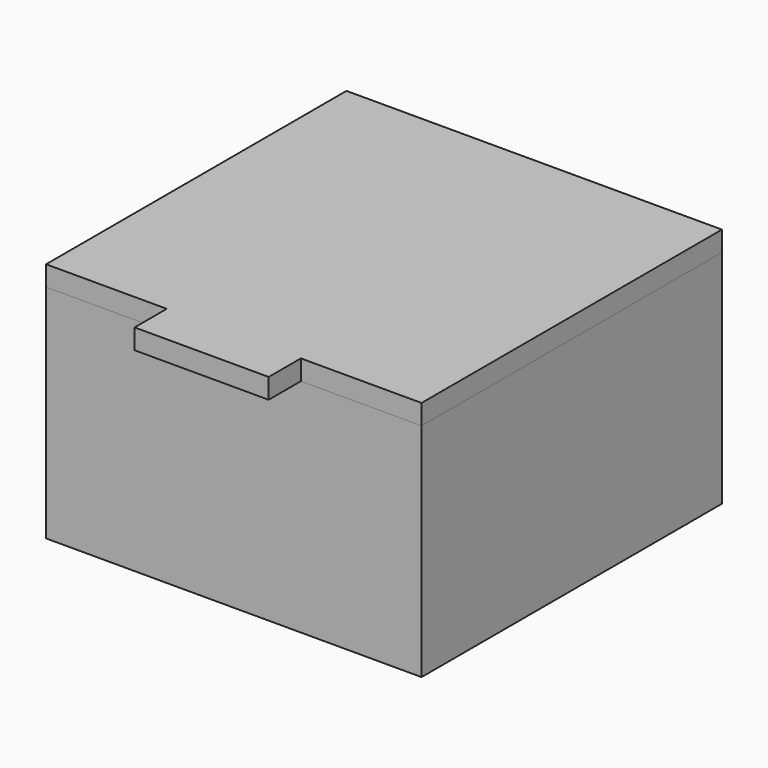
from build123d import *

# Parameters (mm, degrees)
F0_W     = 28
F0_H     = 28
F0_W_2   = 25
F0_H_2   = 25
F1_DEPTH = 1.5
F2_DEPTH = 15
F3_W     = 24.4
F3_H     = 24.4
F3_W_2   = 21.4
F3_H_2   = 21.4
F4_DEPTH = 2
F3_W_3   = 28
F3_H_3   = 28
F3_W_4   = 25
F3_H_4   = 25
F5_DEPTH = 1.5
F6_W     = 10
F6_H     = 1.5
F7_DEPTH = 3


with BuildPart() as f1:
    # F0 (on Top) → F1 (new body)
    with BuildSketch(Plane.XY):
        Rectangle(F0_W, F0_H)
        Rectangle(F0_W_2, F0_H_2, mode=Mode.SUBTRACT)
        Rectangle(F0_W_2, F0_H_2)
    extrude(amount=-F1_DEPTH)

    # F0 (on Top) → F2 (join)
    with BuildSketch(Plane.XY):
        Rectangle(F0_W, F0_H)
        Rectangle(F0_W_2, F0_H_2, mode=Mode.SUBTRACT)
    extrude(amount=F2_DEPTH)


with BuildPart() as f4:
    # F3 (on face) → F4 (new body)
    with BuildSketch(Plane.XY.offset(15)):
        Rectangle(F3_W, F3_H)
        Rectangle(F3_W_2, F3_H_2, mode=Mode.SUBTRACT)
    extrude(amount=-F4_DEPTH)

    # F3 (on face) → F5 (join)
    with BuildSketch(Plane.XY.offset(15)):
        Rectangle(F3_W_3, F3_H_3)
        Rectangle(F3_W_4, F3_H_4, mode=Mode.SUBTRACT)
        Rectangle(F3_W_4, F3_H_4)
        Rectangle(F3_W, F3_H, mode=Mode.SUBTRACT)
        Rectangle(F3_W, F3_H)
        Rectangle(F3_W_2, F3_H_2, mode=Mode.SUBTRACT)
        Rectangle(F3_W_2, F3_H_2)
    extrude(amount=F5_DEPTH)

    # F6 (on face) → F7 (join)
    with BuildSketch(Plane.XZ.offset(14)):
        with Locations((0, 15.75)):
            Rectangle(F6_W, F6_H)
    extrude(amount=F7_DEPTH)


solid = Compound([f1.part, f4.part])
